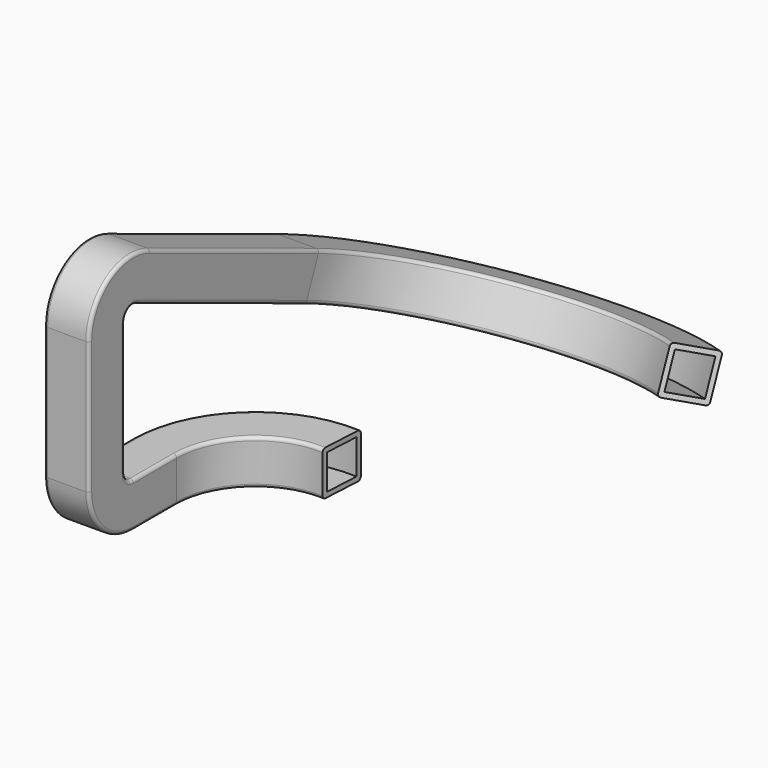
from build123d import *

# Parameters (mm, degrees)
F1_W       = 13.5467974469
F1_H       = 13.5467974469
F1_W_2     = 10.5385975912
F1_H_2     = 10.5385975912
F3_R       = 1
F2_FACE_W  = 10.5385975912
F2_FACE_H  = 10.5385975912
F6_FACE1_W = 10.5385975912
F6_FACE1_H = 10.5385975912


with BuildPart() as f2:
    # F2: sweep along a path in F0
    with BuildLine(Plane.XY) as f2_path:
        ThreePointArc((-30.6053832173, 0), (-21.0397327755, 22.2265410402), (1.6777692664, 30.559361449))
    # F1 (on Front) → F2 (sweep)
    with BuildSketch(Plane.XZ):
        with Locations((-30.6053832173, 0)):
            Rectangle(F1_W, F1_H)
        with Locations((-30.6053832173, 0)):
            Rectangle(F1_W_2, F1_H_2, mode=Mode.SUBTRACT)
    sweep(path=f2_path.line)

    # F3
    f3_edges = [f2.edges().sort_by_distance(p)[0] for p in [
        (-25.696119, 27.145585, 6.773399),
        (-16.383346, 17.307497, 6.773399),
        (-16.383346, 17.307497, -6.773399),
        (-25.696119, 27.145585, -6.773399),
    ]]
    fillet(f3_edges, radius=F3_R)

    # F6: sweep along a path in F5
    with BuildLine(Plane.YZ.offset(-25.3360844217)) as f6_path:
        Line((0, 0), (-16.3940989971, 0))
        ThreePointArc((-16.3940989971, 0), (-23.465166809, 2.9289321881), (-26.3940989971, 10))
        Line((-26.3940989971, 10), (-26.3940989971, 50.0580344714))
        ThreePointArc((-26.3940989971, 50.0580344714), (-21.973146792, 58.3570841581), (-12.6192538566, 59.3181934422))
        Line((-12.6192538566, 59.3181934422), (51.4472291556, 33.2018975093))
    # F2_face (on face) → F6 (sweep)
    with BuildSketch(Plane(origin=(-30.6053832173, 0, 0), x_dir=(1, 0, 0), z_dir=(0, -1, 0))):
        with BuildLine():
            Line((5.7733987235, 6.7733987235), (-5.7733987235, 6.7733987235))
            ThreePointArc((-5.7733987235, 6.7733987235), (-6.4805055046, 6.4805055046), (-6.7733987235, 5.7733987235))
            Line((-6.7733987235, 5.7733987235), (-6.7733987235, -5.7733987235))
            ThreePointArc((-6.7733987235, -5.7733987235), (-6.4805055046, -6.4805055046), (-5.7733987235, -6.7733987235))
            Line((-5.7733987235, -6.7733987235), (5.7733987235, -6.7733987235))
            ThreePointArc((5.7733987235, -6.7733987235), (6.4805055046, -6.4805055046), (6.7733987235, -5.7733987235))
            Line((6.7733987235, -5.7733987235), (6.7733987235, 5.7733987235))
            ThreePointArc((6.7733987235, 5.7733987235), (6.4805055046, 6.4805055046), (5.7733987235, 6.7733987235))
        make_face()
        Rectangle(F2_FACE_W, F2_FACE_H, mode=Mode.SUBTRACT)
    sweep(path=f6_path.line)

    # F8: sweep along a path in F7
    with BuildLine(Plane(origin=(0, 16.9478159309, 41.5750749731), x_dir=(1, 0, 0), z_dir=(0, 0.3774845141, 0.9260158971))) as f8_path:
        ThreePointArc((52.8230853484, 77.5705658045), (1.115810566, 79.5823116094), (-25.3360844217, 35.1077499121))
    # F6_face1 (on face) → F8 (sweep)
    with BuildSketch(Plane(origin=(-30.6053832173, 51.4472291556, 33.2018975093), x_dir=(-1, 0, 0), z_dir=(0, 0.9260158971, -0.3774845141))):
        with BuildLine():
            Line((-5.7733987235, -6.7733987235), (5.7733987235, -6.7733987235))
            ThreePointArc((5.7733987235, -6.7733987235), (6.4805055046, -6.4805055046), (6.7733987235, -5.7733987235))
            Line((6.7733987235, -5.7733987235), (6.7733987235, 5.7733987235))
            ThreePointArc((6.7733987235, 5.7733987235), (6.4805055046, 6.4805055046), (5.7733987235, 6.7733987235))
            Line((5.7733987235, 6.7733987235), (-5.7733987235, 6.7733987235))
            ThreePointArc((-5.7733987235, 6.7733987235), (-6.4805055046, 6.4805055046), (-6.7733987235, 5.7733987235))
            Line((-6.7733987235, 5.7733987235), (-6.7733987235, -5.7733987235))
            ThreePointArc((-6.7733987235, -5.7733987235), (-6.4805055046, -6.4805055046), (-5.7733987235, -6.7733987235))
        make_face()
        Rectangle(F6_FACE1_W, F6_FACE1_H, mode=Mode.SUBTRACT)
    sweep(path=f8_path.line)


solid = f2.part
